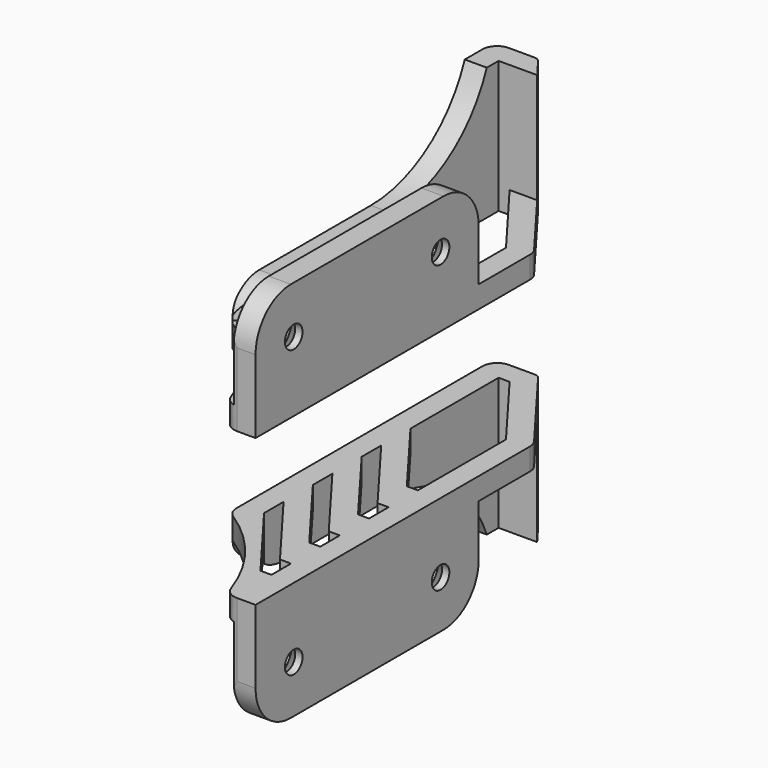
from build123d import *

# Parameters (mm, degrees)
F1_DEPTH     = 3
F2_R         = 1.5
F3_DEPTH     = 3
F4_SIZE      = 2
F6_DEPTH     = 15
F8_DEPTH     = 5
F9_T1_DEPTH  = 42
F9_T3_DEPTH  = 16.3175757864
F9_T5_DEPTH  = 20.6618120859
F9_T7_DEPTH  = 11.030287668
F10_T1_DEPTH = 20.4929080403


# Not quite as in the source:
# - a fillet or chamfer that OpenCascade refuses, or shapes differently, is made with other operations: its cross-section is extruded or revolved along the edge and cut away or added


with BuildPart() as f1:
    # F0 (on Top) → F1 (new body)
    with BuildSketch(Plane.XY):
        with BuildLine():
            Line((6, 30), (0, 30))
            Line((0, 30), (0, -15))
            ThreePointArc((0, -15), (7.1943680268, -21.3926511795), (11.5, -30))
            Line((11.5, -30), (15.5, -30))
            Line((15.5, -30), (15.5, 17.3930741946))
            Line((15.5, 17.3930741946), (6, 30))
        make_face()
        Polygon((3, -9.6013218346), (10.9957448242, -20.2120335985), (12.5, -20.2120335985), (12.5, -23.5353138807), (10.9957448242, -23.5353138807), (3, -12.9246021168), align=None, mode=Mode.SUBTRACT)
        Polygon((10.9957448242, -15.2271131751), (3, -4.6164014112), (3, -1.293121129), (10.9957448242, -11.9038328929), (12.5, -11.9038328929), (12.5, -15.2271131751), align=None, mode=Mode.SUBTRACT)
        Polygon((3, 3.6917992944), (3, 7.0150795766), (10.9957448242, -3.5956321873), (12.5, -3.5956321873), (12.5, -6.9189124695), (10.9957448242, -6.9189124695), align=None, mode=Mode.SUBTRACT)
        Polygon((4.5042551758, 27), (12.5, 16.3892882361), (12.5, 1.3892882361), (10.9957448242, 1.3892882361), (3, 12), (3, 27), align=None, mode=Mode.SUBTRACT)
    extrude(amount=F1_DEPTH)

    # F2 (on face) → F3 (join)
    with BuildSketch(Plane.YZ.offset(15.5)):
        with BuildLine():
            Line((-30, 3), (8, 3))
            Line((8, 3), (8, 10))
            ThreePointArc((8, 10), (6.2426406871, 14.2426406871), (2, 16))
            Line((2, 16), (-24, 16))
            ThreePointArc((-24, 16), (-28.2426406871, 14.2426406871), (-30, 10))
            Line((-30, 10), (-30, 3))
        make_face()
        with Locations((-23.5, 9.5)):
            Circle(F2_R, mode=Mode.SUBTRACT)
        with Locations((1.5, 9.5)):
            Circle(F2_R, mode=Mode.SUBTRACT)
    extrude(amount=-F3_DEPTH)

    # F4
    f4_edges = [f1.edges().sort_by_distance(p)[0] for p in [
        (12.5, -25, 9.5),
        (12.5, 0, 9.5),
    ]]
    chamfer(f4_edges, length=F4_SIZE)

    # F5 (on face) → F6 (join)
    with BuildSketch(Plane.XY.offset(3)):
        Polygon((6, 30), (0, 30), (0, -15), (3, -12.9246021168), (3, 27), (4.5042551758, 27), (8.2606621503, 27), align=None)
    extrude(amount=F6_DEPTH)

    # F7 (on face) → F8 (cut)
    with BuildSketch(Plane(origin=(0, 0, 0), x_dir=(0, -1, 0), z_dir=(-1, 0, 0))):
        with BuildLine():
            Line((-9, 7), (10, 7))
            ThreePointArc((10, 7), (13.2015621187, 5.8769526484), (15, 3))
            Line((15, 3), (15, 18))
            Line((15, 18), (-25, 18))
            ThreePointArc((-25, 18), (-18.7082439195, 10.0152815717), (-9, 7))
        make_face()
    extrude(amount=-F8_DEPTH, mode=Mode.SUBTRACT)

    # F9: fillet of radius 2 on 4 edges, made by hand

    # F9_s2 → F9_t1 (cut)
    with BuildSketch(Plane.XY.offset(-12)):
        with BuildLine():
            ThreePointArc((2, 30), (0.5857864376, 29.4142135624), (0, 28))
            Line((0, 28), (-0.04, 28))
            Line((-0.04, 28), (-0.04, 30.04))
            Line((-0.04, 30.04), (2, 30.04))
            Line((2, 30.04), (2, 30))
        make_face()
    extrude(amount=F9_T1_DEPTH, mode=Mode.SUBTRACT)

    # F9_s4 → F9_t3 (cut)
    with BuildSketch(Plane.XY.offset(-6.6587878932)):
        with BuildLine():
            ThreePointArc((0, -13.8902020178), (0.2412952553, -14.8425452443), (0.9069576211, -15.5650925688))
            Line((0.9069576211, -15.5650925688), (0.8850967735, -15.5985903798))
            ThreePointArc((0.8850967735, -15.5985903798), (0.4352927921, -15.3117343307), (-0.0204351682, -15.0343861004))
            Line((-0.0204351682, -15.0343861004), (-0.04, -15))
            Line((-0.04, -15), (-0.04, -13.8902020178))
            Line((-0.04, -13.8902020178), (0, -13.8902020178))
        make_face()
    extrude(amount=F9_T3_DEPTH, mode=Mode.SUBTRACT)

    # F9_s6 → F9_t5 (cut)
    with BuildSketch(Plane.XY.offset(-8.830906043)):
        with BuildLine():
            ThreePointArc((11.0792645155, -28.6467167409), (11.8085106382, -29.626873302), (12.9718176738, -30))
            Line((12.9718176738, -30), (12.9718176738, -30.04))
            Line((12.9718176738, -30.04), (11.5, -30.04))
            Line((11.5, -30.04), (11.4614875676, -30.0108070601))
            ThreePointArc((11.4614875676, -30.0108070601), (11.2608585475, -29.332304111), (11.0414134523, -28.6596510757))
            Line((11.0414134523, -28.6596510757), (11.0792645155, -28.6467167409))
        make_face()
    extrude(amount=F9_T5_DEPTH, mode=Mode.SUBTRACT)

    # F9_s8 → F9_t7 (cut)
    with BuildSketch(Plane.XY.offset(-4.015143834)):
        with BuildLine():
            ThreePointArc((15.5, 16.7238835556), (15.3966473104, 17.3584928684), (15.0972710201, 17.9275136019))
            Line((15.0972710201, 17.9275136019), (15.1292164405, 17.9515862028))
            Line((15.1292164405, 17.9515862028), (15.54, 17.4064580074))
            Line((15.54, 17.4064580074), (15.54, 16.7238835556))
            Line((15.54, 16.7238835556), (15.5, 16.7238835556))
        make_face()
    extrude(amount=F9_T7_DEPTH, mode=Mode.SUBTRACT)

    # F10: fillet of radius 1 on 1 edges, made by hand

    # F10_s2 → F10_t1 (cut)
    with BuildSketch(Plane.XY.offset(-1.2464540201)):
        with BuildLine():
            ThreePointArc((5.5014183919, 30), (5.9476162051, 29.8949343616), (6.300053902, 29.6018150232))
            Line((6.300053902, 29.6018150232), (6, 30))
            Line((6, 30), (5.5014183919, 30))
        make_face()
    extrude(amount=F10_T1_DEPTH, mode=Mode.SUBTRACT)


with BuildPart() as f11_1:
    # F11: instance of F1
    add(f1.part.mirror(Plane.XY))


with BuildPart() as f1_1:
    # F12: moved
    add(f1.part.moved(Location((0, 0, 10))))


with BuildPart() as f11_1_1:
    # F13: moved
    add(f11_1.part.moved(Location((0, 0, -10))))


solid = Compound([f1_1.part, f11_1_1.part])
